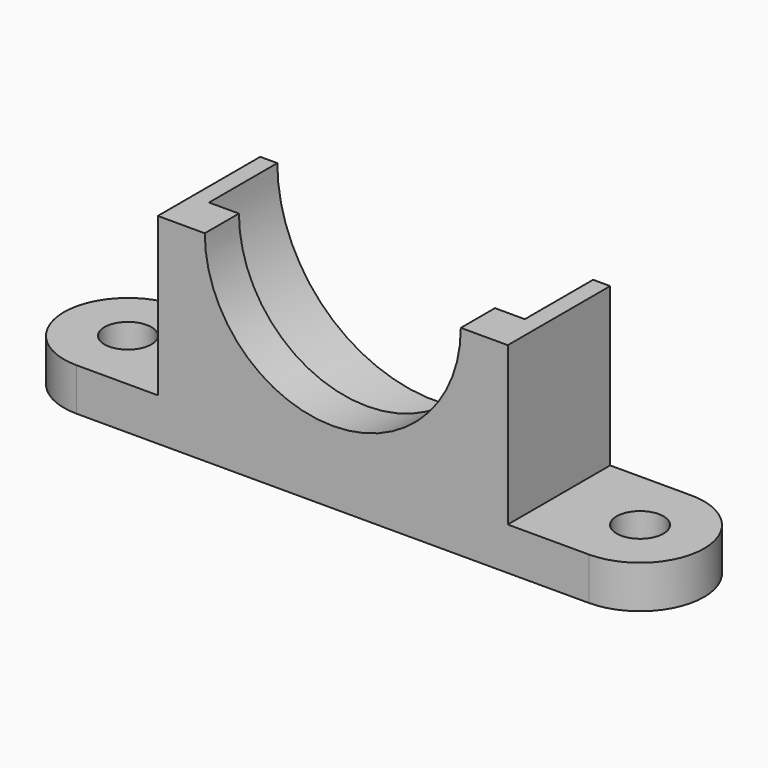
from build123d import *

# Parameters (mm, degrees)
F0_W     = 60
F0_H     = 15
F1_DEPTH = 5
F3_DEPTH = 15
F4_DEPTH = 5
F6_D     = 5.5


with BuildPart() as f1:
    # F0 (on Top) → F1 (new body)
    with BuildSketch(Plane.XY):
        Rectangle(F0_W, F0_H)
        with BuildLine():
            Line((-30, -7.5), (-30, 7.5))
            ThreePointArc((-30, 7.5), (-37.5, 0), (-30, -7.5))
        make_face()
        with BuildLine():
            ThreePointArc((30, -7.5), (37.5, 0), (30, 7.5))
            Line((30, 7.5), (30, -7.5))
        make_face()
    extrude(amount=F1_DEPTH)

    # F2 (on face) → F3 (join)
    with BuildSketch(Plane.XZ.offset(7.5)):
        with BuildLine():
            Line((20.5, 23.5), (18.5, 23.5))
            ThreePointArc((18.5, 23.5), (13.0814754325, 10.4185245286), (-5.51e-08, 5))
            Line((-5.51e-08, 5), (8.8317608663, 5))
            ThreePointArc((8.8317608663, 5), (17.3392776343, 12.5638466031), (20.5, 23.5))
        make_face()
        with BuildLine():
            ThreePointArc((-5.51e-08, 5), (-13.0814754714, 10.4185245675), (-18.5, 23.5))
            Line((-18.5, 23.5), (-20.5, 23.5))
            ThreePointArc((-20.5, 23.5), (-17.3392776343, 12.5638466031), (-8.8317608663, 5))
            Line((-8.8317608663, 5), (-5.51e-08, 5))
        make_face()
        with BuildLine():
            Line((20.5, 5), (20.5, 23.5))
            ThreePointArc((20.5, 23.5), (17.3392776343, 12.5638466031), (8.8317608663, 5))
            Line((8.8317608663, 5), (20.5, 5))
        make_face()
        with BuildLine():
            ThreePointArc((-8.8317608663, 5), (-17.3392776343, 12.5638466031), (-20.5, 23.5))
            Line((-20.5, 23.5), (-20.5, 5))
            Line((-20.5, 5), (-8.8317608663, 5))
        make_face()
    extrude(amount=-F3_DEPTH)

    # F2 (on face) → F4 (join)
    with BuildSketch(Plane.XZ.offset(7.5)):
        with BuildLine():
            ThreePointArc((-5.51e-08, 5), (13.0814754325, 10.4185245286), (18.5, 23.5))
            Line((18.5, 23.5), (15, 23.5))
            ThreePointArc((15, 23.5), (0, 8.5), (-15, 23.5))
            Line((-15, 23.5), (-18.5, 23.5))
            ThreePointArc((-18.5, 23.5), (-13.0814754714, 10.4185245675), (-5.51e-08, 5))
        make_face()
    extrude(amount=-F4_DEPTH)

    # F6 (through all)
    with Locations(Plane.XY.offset(5)):
        with Locations((30, 0), (-30, 0)):
            Hole(F6_D / 2)


solid = f1.part
